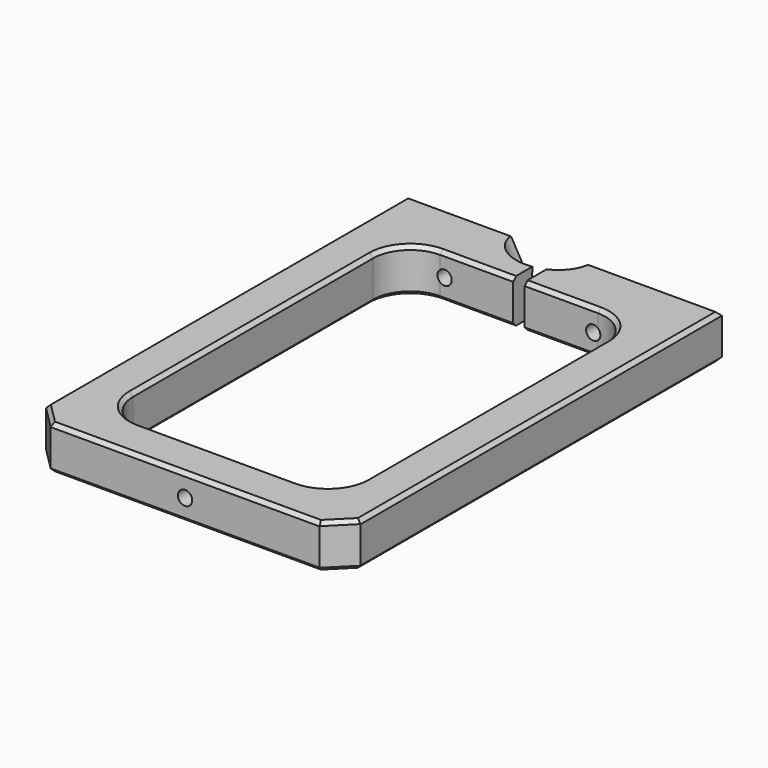
from build123d import *

# Parameters (mm, degrees)
F0_W         = 34.925
F0_H         = 52.705
F1_DEPTH     = 9.7155
F2_W         = 25.781
F2_H         = 43.18
F2_H_2       = 40.005
F3_DEPTH     = 25.4
F4_R         = 8.255
F5_SIZE      = 0.8255
F6_R         = 1.5875
F7_DEPTH     = 25.4
F8_T1_DEPTH  = 34.1927991577
F9_SIZE      = 0.79375
F10_R        = 1.5875
F11_DEPTH    = 25.4
F13_R        = 7.493
F14_DEPTH    = 50.8
F15_T1_DEPTH = 13.2391086204
F15_T3_DEPTH = 13.2391086204
F16_W        = 2.54
F16_H        = 15.24
F17_DEPTH    = 25.4


# Not quite as in the source:
# - a fillet or chamfer that OpenCascade refuses, or shapes differently, is made with other operations: its cross-section is extruded or revolved along the edge and cut away or added
# - a feature names something its author has since deleted; it is built from what else it names


with BuildPart() as f1:
    # F0 (on Top) → F1 (new body)
    with BuildSketch(Plane.XY):
        with Locations((-17.4625, -26.3525)):
            Rectangle(F0_W, F0_H)
        with Locations((-17.4625, 26.3525)):
            Rectangle(F0_W, F0_H)
        Polygon((0, 52.705), (0, 0), (0, -52.705), (34.925, -52.705), (34.925, 0), (34.925, 52.705), align=None)
    extrude(amount=F1_DEPTH)

    # F2 (on face) → F3 (cut)
    with BuildSketch(Plane.XY.offset(9.7155)):
        with Locations((-12.8905, -21.59)):
            Rectangle(F2_W, F2_H)
        with Locations((-12.8905, 20.0025)):
            Rectangle(F2_W, F2_H_2)
        with Locations((12.8905, -21.59)):
            Rectangle(F2_W, F2_H)
        with Locations((12.8905, 20.0025)):
            Rectangle(F2_W, F2_H_2)
    extrude(amount=-F3_DEPTH, mode=Mode.SUBTRACT)

    # F4
    f4_edges = [f1.edges().sort_by_distance(p)[0] for p in [
        (-25.781, 40.005, 4.85775),
        (25.781, 40.005, 4.85775),
        (-25.781, -43.18, 4.85775),
        (25.781, -43.18, 4.85775),
    ]]
    fillet(f4_edges, radius=F4_R)

    # F5
    f5_edges = [f1.edges().sort_by_distance(p)[0] for p in [
        (-34.925, 0, 9.7155),
        (-25.781, -1.5875, 9.7155),
        (34.925, 0, 9.7155),
        (0, -52.705, 9.7155),
        (0, 52.705, 9.7155),
        (-34.925, 0, 0),
        (0, -52.705, 0),
        (34.925, 0, 0),
        (25.781, -1.5875, 0),
        (0, 52.705, 0),
        (-25.781, -1.5875, 0),
        (-23.363166, 37.587166, 0),
        (-23.363166, -40.762166, 0),
        (0, 40.005, 0),
        (0, -43.18, 0),
        (23.363166, 37.587166, 0),
        (23.363166, -40.762166, 0),
        (-23.363166, 37.587166, 9.7155),
        (-23.363166, -40.762166, 9.7155),
        (0, 40.005, 9.7155),
        (0, -43.18, 9.7155),
        (23.363166, 37.587166, 9.7155),
        (23.363166, -40.762166, 9.7155),
        (25.781, -1.5875, 9.7155),
    ]]
    chamfer(f5_edges, length=F5_SIZE)

    # F6 (on face) → F7 (cut)
    with BuildSketch(Plane(origin=(0, 52.705, 0), x_dir=(-1, 0, 0), z_dir=(0, 1, 0))):
        with Locations((-16.51, 4.7625)):
            Circle(F6_R)
        with Locations((16.51, 4.7625)):
            Circle(F6_R)
    extrude(amount=-F7_DEPTH, mode=Mode.SUBTRACT)

    # F8: chamfer of 5.08 on 2 edges, made by hand

    # F8_s2 → F8_t1 (cut)
    with BuildSketch(Plane.XY.offset(-12.2386495789)):
        Polygon((-34.925, -47.625), (-29.845, -52.705), (-34.925, -52.705), align=None)
        Polygon((29.845, -52.705), (34.925, -47.625), (34.925, -52.705), align=None)
    extrude(amount=F8_T1_DEPTH, mode=Mode.SUBTRACT)

    # F9
    f9_edges = [f1.edges().sort_by_distance(p)[0] for p in [
        (-32.385, -50.165, 0),
        (32.385, -50.165, 0),
        (32.385, -50.165, 9.7155),
        (-32.385, -50.165, 9.7155),
    ]]
    chamfer(f9_edges, length=F9_SIZE)

    # F10 (on face) → F11 (cut)
    with BuildSketch(Plane.XZ.offset(52.705)):
        with Locations((0, 4.7625)):
            Circle(F10_R)
    extrude(amount=-F11_DEPTH, mode=Mode.SUBTRACT)

    # F13 (on face) + F2 (on face) → F14 (cut)
    with BuildSketch(Plane(origin=(8.524875, 0, -14.7655166282), x_dir=(0.8660254038, 0, 0.5), z_dir=(0.5, 0, -0.8660254038))):
        with Locations((2.460086914, -52.705)):
            Circle(F13_R)
    with BuildSketch(Plane.XY.offset(9.7155)):
        with Locations((-12.8905, -21.59)):
            Rectangle(F2_W, F2_H)
        with Locations((-12.8905, 20.0025)):
            Rectangle(F2_W, F2_H_2)
        with Locations((12.8905, -21.59)):
            Rectangle(F2_W, F2_H)
        with Locations((12.8905, 20.0025)):
            Rectangle(F2_W, F2_H_2)
    extrude(amount=-F14_DEPTH, dir=(0.5, 0, -0.8660254038), mode=Mode.SUBTRACT)

    # F15: chamfer of 0.8001 on 2 edges, made by hand

    # F15_s2 → F15_t1 (cut)
    with BuildSketch(Plane(origin=(3.3783625895, 0, -5.8514956514), x_dir=(0, 1, 0), z_dir=(-0.5, 0, 0.8660254038))):
        with BuildLine():
            Line((52.705, -10.7145007393), (51.9820918836, -9.9181330962))
            ThreePointArc((51.9820918836, -9.9181330962), (52.3317918419, -9.9437868459), (52.705, -9.953086914))
            Line((52.705, -9.953086914), (52.705, -10.7145007393))
        make_face()
    extrude(amount=F15_T1_DEPTH, mode=Mode.SUBTRACT)

    # F15_s4 → F15_t3 (cut)
    with BuildSketch(Plane(origin=(-7.5672772878, 0, 13.1069087374), x_dir=(0, 1, 0), z_dir=(0.5, 0, -0.8660254038))):
        with BuildLine():
            Line((52.705, -5.7943269113), (51.9820918836, -4.9979592682))
            ThreePointArc((51.9820918836, -4.9979592682), (52.3317918419, -5.0236130179), (52.705, -5.032913086))
            Line((52.705, -5.032913086), (52.705, -5.7943269113))
        make_face()
    extrude(amount=F15_T3_DEPTH, mode=Mode.SUBTRACT)

    # F16 (on face) → F17 (cut)
    with BuildSketch(Plane.XZ.offset(-40.005)):
        with Locations((0, 5.08)):
            Rectangle(F16_W, F16_H)
    extrude(amount=-F17_DEPTH, mode=Mode.SUBTRACT)


solid = f1.part
